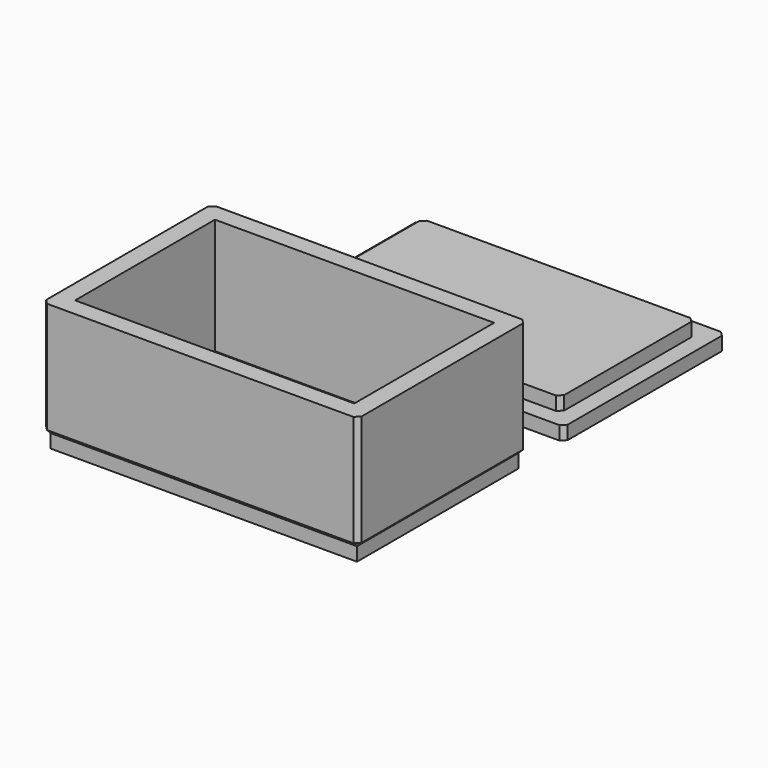
from build123d import *

# Parameters (mm, degrees)
F0_W      = 27
F0_H      = 17.8
F1_DEPTH  = 1.2
F2_W      = 27.8
F2_H      = 18.6
F2_W_2    = 27
F2_H_2    = 17.8
F2_W_3    = 24.6
F2_H_3    = 15.4
F3_DEPTH  = 10.2
F4_W      = 24
F4_H      = 14.8
F5_DEPTH  = 1.2
F6_SIZE   = 0.39999
F6_2_SIZE = 0.39999


# Not quite as in the source:
# - a fillet or chamfer is up to 0.001 mm smaller than in the source, because OpenCascade refuses the exact size


with BuildPart() as f1:
    # F0 (on Top) → F1 (new body)
    with BuildSketch(Plane.XY):
        Rectangle(F0_W, F0_H)
    extrude(amount=F1_DEPTH)

    # F2 (on face) → F3 (join)
    with BuildSketch(Plane.XY.offset(1.2)):
        Rectangle(F2_W, F2_H)
        Rectangle(F2_W_2, F2_H_2, mode=Mode.SUBTRACT)
        Rectangle(F2_W_2, F2_H_2)
        Rectangle(F2_W_3, F2_H_3, mode=Mode.SUBTRACT)
    extrude(amount=F3_DEPTH)

    # F6 (size 0.4 in the source; OpenCascade refuses exactly that, so slightly less here)
    f6_edges = [f1.edges().sort_by_distance(p)[0] for p in [
        (-13.9, 0, 1.2),
        (-13.9, -9.3, 6.3),
        (-13.9, 9.3, 6.3),
        (13.9, -9.3, 6.3),
        (13.9, 0, 1.2),
        (13.9, 9.3, 6.3),
        (0, 9.3, 1.2),
        (0, -9.3, 1.2),
    ]]
    chamfer(f6_edges, length=F6_SIZE)


with BuildPart() as f1b:
    # F0 (on Top) → F1, piece 2 (new body)
    with BuildSketch(Plane.XY):
        with Locations((0, 22.8)):
            Rectangle(F0_W, F0_H)
    extrude(amount=F1_DEPTH)

    # F4 (on face) → F5 (join)
    with BuildSketch(Plane.XY.offset(1.2)):
        with Locations((0, 22.8)):
            Rectangle(F4_W, F4_H)
    extrude(amount=F5_DEPTH)

    # F6#2 (size 0.4 in the source; OpenCascade refuses exactly that, so slightly less here)
    f6_2_edges = [f1b.edges().sort_by_distance(p)[0] for p in [
        (13.5, 31.7, 0.6),
        (12, 30.2, 1.8),
        (12, 15.4, 1.8),
        (13.5, 13.9, 0.6),
        (-13.5, 31.7, 0.6),
        (-12, 30.2, 1.8),
        (-13.5, 13.9, 0.6),
        (-12, 15.4, 1.8),
    ]]
    chamfer(f6_2_edges, length=F6_2_SIZE)


solid = Compound([f1.part, f1b.part])
